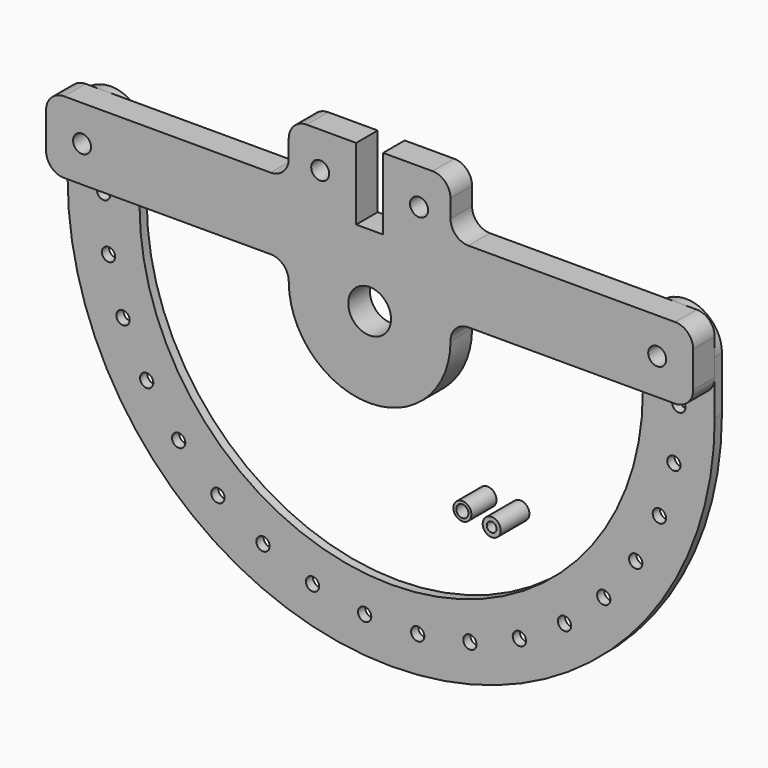
from build123d import *

# Parameters (mm, degrees)
F1_R     = 7.540625
F1_R_2   = 3.175
F2_DEPTH = 9.525
F0_R     = 2.3495
F0_R_2   = 3.175
F3_DEPTH = 3.175
F4_R     = 3.175
F5_DEPTH = 12.7
F6_DEPTH = 11.1125
F7_D     = 3.4544
F8_D     = 4.318


# Not quite as in the source:
# - a length typed as a fraction of an inch, garbled in the dataset ("3 / 203.2 mm" for 3/8 in), is restored


with BuildPart() as f2:
    # F1 (on Front) → F2 (new body)
    with BuildSketch(Plane.XZ):
        with BuildLine():
            ThreePointArc((-28.575, 0), (0, -28.575), (28.575, 0))
            ThreePointArc((28.575, 0), (30.4348719395, 4.4901280605), (34.925, 6.35))
            Line((34.925, 6.35), (107.95, 6.35))
            ThreePointArc((107.95, 6.35), (112.4401280605, 8.2098719395), (114.3, 12.7))
            Line((114.3, 12.7), (114.3, 25.4))
            ThreePointArc((114.3, 25.4), (112.4401280605, 29.8901280605), (107.95, 31.75))
            Line((107.95, 31.75), (34.925, 31.75))
            ThreePointArc((34.925, 31.75), (30.4348719395, 33.6098719395), (28.575, 38.1))
            Line((28.575, 38.1), (28.575, 44.45))
            ThreePointArc((28.575, 44.45), (26.7151280605, 48.9401280605), (22.225, 50.8))
            Line((22.225, 50.8), (4.7625, 50.8))
            Line((4.7625, 50.8), (4.7625, 25.4))
            Line((4.7625, 25.4), (-4.7625, 25.4))
            Line((-4.7625, 25.4), (-4.7625, 50.8))
            Line((-4.7625, 50.8), (-22.225, 50.8))
            ThreePointArc((-22.225, 50.8), (-26.7151280605, 48.9401280605), (-28.575, 44.45))
            Line((-28.575, 44.45), (-28.575, 38.1))
            ThreePointArc((-28.575, 38.1), (-30.4348719395, 33.6098719395), (-34.925, 31.75))
            Line((-34.925, 31.75), (-107.95, 31.75))
            ThreePointArc((-107.95, 31.75), (-112.4401280605, 29.8901280605), (-114.3, 25.4))
            Line((-114.3, 25.4), (-114.3, 12.7))
            ThreePointArc((-114.3, 12.7), (-112.4401280605, 8.2098719395), (-107.95, 6.35))
            Line((-107.95, 6.35), (-34.925, 6.35))
            ThreePointArc((-34.925, 6.35), (-30.4348719395, 4.4901280605), (-28.575, 0))
        make_face()
        Circle(F1_R, mode=Mode.SUBTRACT)
        with Locations((-101.6, 19.05)):
            Circle(F1_R_2, mode=Mode.SUBTRACT)
        with Locations((-17.4625, 38.1)):
            Circle(F1_R_2, mode=Mode.SUBTRACT)
        with Locations((101.6, 19.05)):
            Circle(F1_R_2, mode=Mode.SUBTRACT)
        with Locations((17.4625, 38.1)):
            Circle(F1_R_2, mode=Mode.SUBTRACT)
    extrude(amount=F2_DEPTH)


with BuildPart() as f3:
    # F0 (on Front) → F3 (new body)
    with BuildSketch(Plane.XZ):
        with BuildLine():
            Line((-114.3, 19.05), (-114.3, 0))
            ThreePointArc((-114.3, 0), (0, -114.3), (114.3, 0))
            Line((114.3, 0), (114.3, 19.05))
            ThreePointArc((114.3, 19.05), (101.6, 31.75), (88.9, 19.05))
            Line((88.9, 19.05), (88.9, 0))
            ThreePointArc((88.9, 0), (0, -88.9), (-88.9, 0))
            Line((-88.9, 0), (-88.9, 19.05))
            ThreePointArc((-88.9, 19.05), (-101.6, 31.75), (-114.3, 19.05))
        make_face()
        with Locations((-61.2276790561, -81.0785502917)):
            Circle(F0_R, mode=Mode.SUBTRACT)
        with Locations((-27.8041597913, -97.7214853464)):
            Circle(F0_R, mode=Mode.SUBTRACT)
        with Locations((-9.3744653215, -101.1665923116)):
            Circle(F0_R, mode=Mode.SUBTRACT)
        with Locations((-45.2870169469, -90.9485904017)):
            Circle(F0_R, mode=Mode.SUBTRACT)
        with Locations((-75.0833059896, -68.4474773945)):
            Circle(F0_R, mode=Mode.SUBTRACT)
        with Locations((-86.3820609901, -53.4855077483)):
            Circle(F0_R, mode=Mode.SUBTRACT)
        with Locations((9.3744653215, -101.1665923116)):
            Circle(F0_R, mode=Mode.SUBTRACT)
        with Locations((27.8041597913, -97.7214853464)):
            Circle(F0_R, mode=Mode.SUBTRACT)
        with Locations((45.2870169469, -90.9485904017)):
            Circle(F0_R, mode=Mode.SUBTRACT)
        with Locations((61.2276790561, -81.0785502917)):
            Circle(F0_R, mode=Mode.SUBTRACT)
        with Locations((75.0833059896, -68.4474773945)):
            Circle(F0_R, mode=Mode.SUBTRACT)
        with Locations((86.3820609901, -53.4855077483)):
            Circle(F0_R, mode=Mode.SUBTRACT)
        with Locations((-94.7391785075, -36.7021532846)):
            Circle(F0_R, mode=Mode.SUBTRACT)
        with Locations((-99.8700669279, -18.6689510102)):
            Circle(F0_R, mode=Mode.SUBTRACT)
        with Locations((-101.6, 0)):
            Circle(F0_R, mode=Mode.SUBTRACT)
        with Locations((-101.6, 19.05)):
            Circle(F0_R_2, mode=Mode.SUBTRACT)
        with Locations((94.7391785075, -36.7021532846)):
            Circle(F0_R, mode=Mode.SUBTRACT)
        with Locations((99.8700669279, -18.6689510102)):
            Circle(F0_R, mode=Mode.SUBTRACT)
        with Locations((101.6, 0)):
            Circle(F0_R, mode=Mode.SUBTRACT)
        with Locations((101.6, 19.05)):
            Circle(F0_R_2, mode=Mode.SUBTRACT)
    extrude(amount=-F3_DEPTH)


with BuildPart() as f5:
    # F4 (on Front) → F5 (new body)
    with BuildSketch(Plane.XZ):
        with Locations((45.6634163857, -51.0011874139)):
            Circle(F4_R)
    extrude(amount=F5_DEPTH)

    # F7 (through all)
    with Locations(Plane(origin=(0, 0, 0), x_dir=(1, 0, 0), z_dir=(0, 1, 0))):
        with Locations((45.6634163857, 51.0011874139)):
            Hole(F7_D / 2)


with BuildPart() as f6:
    # F4 (on Front) → F6 (new body)
    with BuildSketch(Plane.XZ):
        with Locations((34.0374670923, -50.4689142108)):
            Circle(F4_R)
    extrude(amount=F6_DEPTH)

    # F8 (through all)
    with Locations(Plane(origin=(0, 0, 0), x_dir=(1, 0, 0), z_dir=(0, 1, 0))):
        with Locations((34.0374670923, 50.4689142108)):
            Hole(F8_D / 2)


solid = Compound([f2.part, f3.part, f5.part, f6.part])
